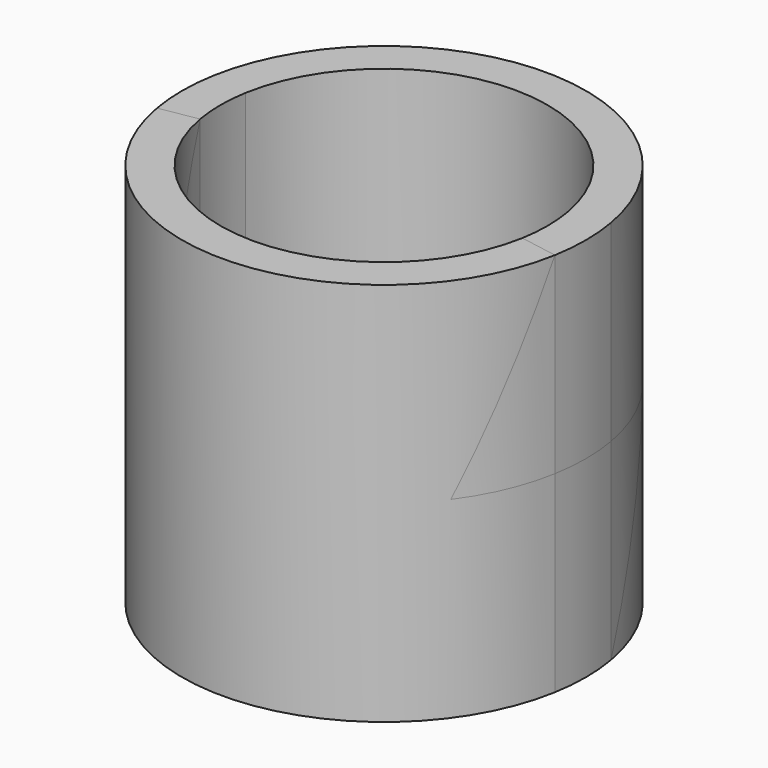
from build123d import *

# Parameters (mm, degrees)
F3_DEPTH  = 15
F4_DEPTH  = 15
F5_SIZE2  = 14.99999
F5_SIZE   = 6.994605
F6_ANGLE  = 180
F9_ANGLE  = 180
F11_ANGLE = 180


# Not quite as in the source:
# - a fillet or chamfer is up to 0.001 mm smaller than in the source, because OpenCascade refuses the exact size


with BuildPart() as f3:
    # F2 (on Top) → F3 (new body)
    with BuildSketch(Plane.XY):
        with BuildLine():
            ThreePointArc((12.5562988509, 2.2140142653), (12.75, 0), (12.5562988509, -2.2140142653))
            Line((12.5562988509, -2.2140142653), (15.5107221099, -2.7349587983))
            ThreePointArc((15.5107221099, -2.7349587983), (15.75, 0), (15.5107221099, 2.7349587983))
            Line((15.5107221099, 2.7349587983), (12.5562988509, 2.2140142653))
        make_face()
        with BuildLine():
            ThreePointArc((12.5562988509, -2.2140142653), (0, -12.75), (-12.5562988509, -2.2140142653))
            Line((-12.5562988509, -2.2140142653), (-15.5107221099, -2.7349587983))
            ThreePointArc((-15.5107221099, -2.7349587983), (0, -15.75), (15.5107221099, -2.7349587983))
            Line((15.5107221099, -2.7349587983), (12.5562988509, -2.2140142653))
        make_face()
        with BuildLine():
            Line((-15.5107221099, -2.7349587983), (-12.5562988509, -2.2140142653))
            ThreePointArc((-12.5562988509, -2.2140142653), (-12.75, 0), (-12.5562988509, 2.2140142653))
            Line((-12.5562988509, 2.2140142653), (-15.5107221099, 2.7349587983))
            ThreePointArc((-15.5107221099, 2.7349587983), (-15.75, 0), (-15.5107221099, -2.7349587983))
        make_face()
        with BuildLine():
            Line((-15.5107221099, 2.7349587983), (-12.5562988509, 2.2140142653))
            ThreePointArc((-12.5562988509, 2.2140142653), (0, 12.75), (12.5562988509, 2.2140142653))
            Line((12.5562988509, 2.2140142653), (15.5107221099, 2.7349587983))
            ThreePointArc((15.5107221099, 2.7349587983), (0, 15.75), (-15.5107221099, 2.7349587983))
        make_face()
    extrude(amount=F3_DEPTH)


with BuildPart() as f4:
    # F2 (on Top) → F4 (new body)
    with BuildSketch(Plane.XY):
        with BuildLine():
            Line((-15.5107221099, 2.7349587983), (-12.5562988509, 2.2140142653))
            ThreePointArc((-12.5562988509, 2.2140142653), (0, 12.75), (12.5562988509, 2.2140142653))
            Line((12.5562988509, 2.2140142653), (15.5107221099, 2.7349587983))
            ThreePointArc((15.5107221099, 2.7349587983), (0, 15.75), (-15.5107221099, 2.7349587983))
        make_face()
    extrude(amount=-F4_DEPTH)

    # F5 (size 6.9946148723 and 15 in the source; OpenCascade refuses exactly that, so slightly less here)
    f5_edges = [f4.edges().sort_by_distance(p)[0] for p in [
        (-14.03351, 2.474487, -15),
        (14.03351, 2.474487, -15),
    ]]
    f5_side = f4.faces().sort_by_distance((0, 15.41154, -15))[0]
    chamfer(f5_edges, length=F5_SIZE, length2=F5_SIZE2, reference=f5_side)


with BuildPart() as f4_1:
    # F6: moved
    add(f4.part.rotate(Axis((0, -13.477217406, 0), (0, -1, 0)), F6_ANGLE))


with BuildPart() as f3_1:
    add(f3.part)

    # F7: cut F4
    add(f4_1.part, mode=Mode.SUBTRACT)


with BuildPart() as f4_2:
    # F9: moved
    add(f4_1.part.rotate(Axis((-13.7243829668, 0, 15), (-1, 0, 0)), F9_ANGLE))


with BuildPart() as f3_2:
    add(f3_1.part)

    # F10: union F4
    add(f4_2.part)


with BuildPart() as f11_1:
    # F11: copy of F3
    add(f3_2.part.rotate(Axis((-13.7243829668, 0, 15), (-1, 0, 0)), F11_ANGLE))


solid = Compound([f3_2.part, f11_1.part])
